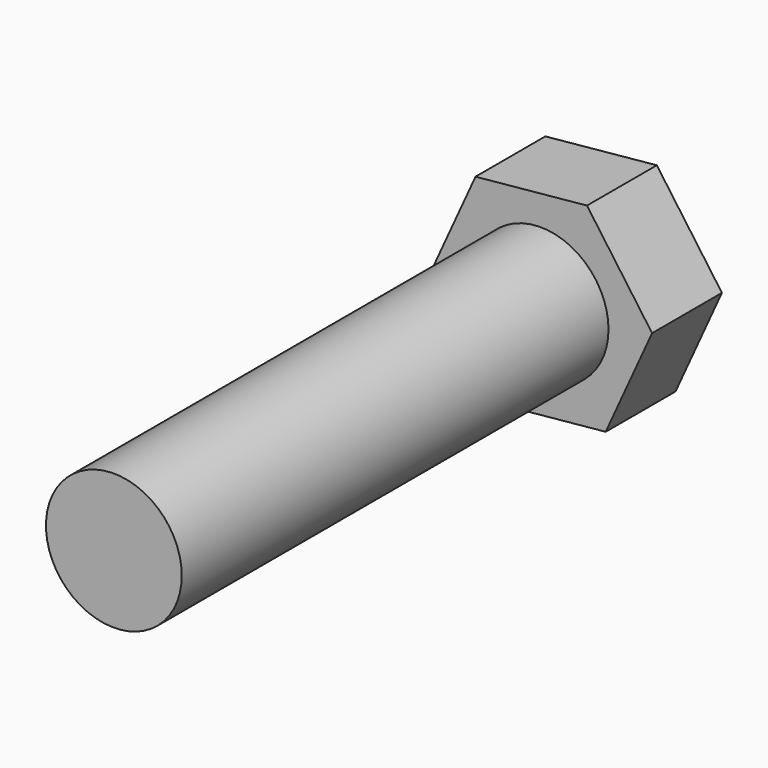
from build123d import *

# Parameters (mm, degrees)
F1_DEPTH = 7.14375
F2_R     = 5.55625
F3_DEPTH = 50.8


# Not quite as in the source:
# - a length typed as a fraction of an inch, garbled in the dataset ("3 / 203.2 mm" for 3/8 in), is restored


with BuildPart() as f1:
    # F0 (on Front) → F1 (new body)
    with BuildSketch(Plane.XZ):
        Polygon((9.122660006, 0.8844674945), (3.795358684, 8.3426890625), (-5.327301322, 7.458221568), (-9.122660006, -0.8844674945), (-3.795358684, -8.3426890625), (5.327301322, -7.458221568), align=None)
    extrude(amount=F1_DEPTH)

    # F2 (on Front) → F3 (join)
    with BuildSketch(Plane.XZ):
        Circle(F2_R)
    extrude(amount=F3_DEPTH)


solid = f1.part
